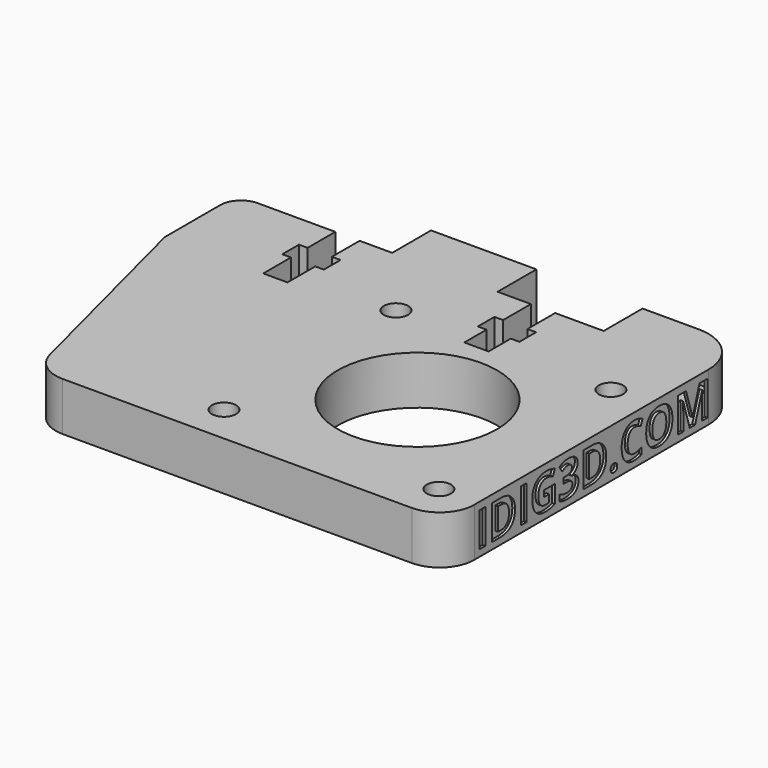
from build123d import *

# Parameters (mm, degrees)
F0_R         = 1.75
F0_R_2       = 11.5
F0_W         = 15.2
F0_H         = 7
F1_DEPTH     = 7
F2_TEXT_SIZE = 6.9444444444
F3_DEPTH     = 0.4
F4_DEPTH     = 1


# Not quite as in the source:
# - a feature names something its author has since deleted; it is built from what else it names
# - Text() gives the source's letters only with a copy of the font that has no kerning and outlines rounded to 1/6400 em; it was checked with that copy


with BuildPart() as f1:
    # F0 (on Top) → F1 (new body)
    with BuildSketch(Plane.XY):
        with BuildLine():
            Line((-19.8, 23.6), (-31, 23.6))
            ThreePointArc((-31, 23.6), (-33.1213203436, 22.7213203436), (-34, 20.6))
            Line((-34, 20.6), (-34, 10.6))
            Line((-34, 10.6), (-26.2072974785, -19.8400206007))
            ThreePointArc((-26.2072974785, -19.8400206007), (-24.4294361355, -22.5496900514), (-21.3635025912, -23.6))
            Line((-21.3635025912, -23.6), (29, -23.6))
            ThreePointArc((29, -23.6), (32.5355339059, -22.1355339059), (34, -18.6))
            Line((34, -18.6), (34, 23.6))
            Line((34, 23.6), (18.9, 23.6))
            Line((18.9, 23.6), (11.9, 23.6))
            Line((11.9, 23.6), (11.9, 18.6))
            Line((11.9, 18.6), (13.15, 18.6))
            Line((13.15, 18.6), (13.15, 15.6))
            Line((13.15, 15.6), (11.9, 15.6))
            Line((11.9, 15.6), (11.9, 10.6))
            Line((11.9, 10.6), (8.4, 10.6))
            Line((8.4, 10.6), (8.4, 15.6))
            Line((8.4, 15.6), (7.15, 15.6))
            Line((7.15, 15.6), (7.15, 18.6))
            Line((7.15, 18.6), (8.4, 18.6))
            Line((8.4, 18.6), (8.4, 23.6))
            Line((8.4, 23.6), (3.6, 23.6))
            Line((3.6, 23.6), (-11.6, 23.6))
            Line((-11.6, 23.6), (-16.3, 23.6))
            Line((-16.3, 23.6), (-16.3, 18.6))
            Line((-16.3, 18.6), (-15.05, 18.6))
            Line((-15.05, 18.6), (-15.05, 15.6))
            Line((-15.05, 15.6), (-16.3, 15.6))
            Line((-16.3, 15.6), (-16.3, 10.6))
            Line((-16.3, 10.6), (-19.8, 10.6))
            Line((-19.8, 10.6), (-19.8, 15.6))
            Line((-19.8, 15.6), (-21.05, 15.6))
            Line((-21.05, 15.6), (-21.05, 18.6))
            Line((-21.05, 18.6), (-19.8, 18.6))
            Line((-19.8, 18.6), (-19.8, 23.6))
        make_face()
        with Locations((-2.5, -18.1)):
            Circle(F0_R, mode=Mode.SUBTRACT)
        with Locations((28.5, -18.1)):
            Circle(F0_R, mode=Mode.SUBTRACT)
        with Locations((13, -2.6)):
            Circle(F0_R_2, mode=Mode.SUBTRACT)
        with Locations((-2.5, 12.9)):
            Circle(F0_R, mode=Mode.SUBTRACT)
        with Locations((28.5, 12.9)):
            Circle(F0_R, mode=Mode.SUBTRACT)
        with Locations((-4, 27.1)):
            Rectangle(F0_W, F0_H)
        with BuildLine():
            Line((18.9, 30.6), (18.9, 23.6))
            Line((18.9, 23.6), (34, 23.6))
            ThreePointArc((34, 23.6), (31.9497474683, 28.5497474683), (27, 30.6))
            Line((27, 30.6), (18.9, 30.6))
        make_face()
    extrude(amount=F1_DEPTH)

    # F2 (on face) → F3 (cut)
    with BuildSketch(Plane.YZ.offset(34)):
        with Locations((-18.2872552812, 0.9590099761)):
            Text('IDIG3D.COM', F2_TEXT_SIZE, font='Open Sans', font_style=FontStyle.BOLD, text_align=(TextAlign.LEFT, TextAlign.BOTTOM))
    extrude(amount=-F3_DEPTH, mode=Mode.SUBTRACT)

    # F4 (add): a face of the model
    f4_faces = [f1.faces().sort_by_distance(p)[0] for p in [
        (10.15, 10.6, 3.5),
    ]]
    extrude(f4_faces, amount=F4_DEPTH)


solid = f1.part
